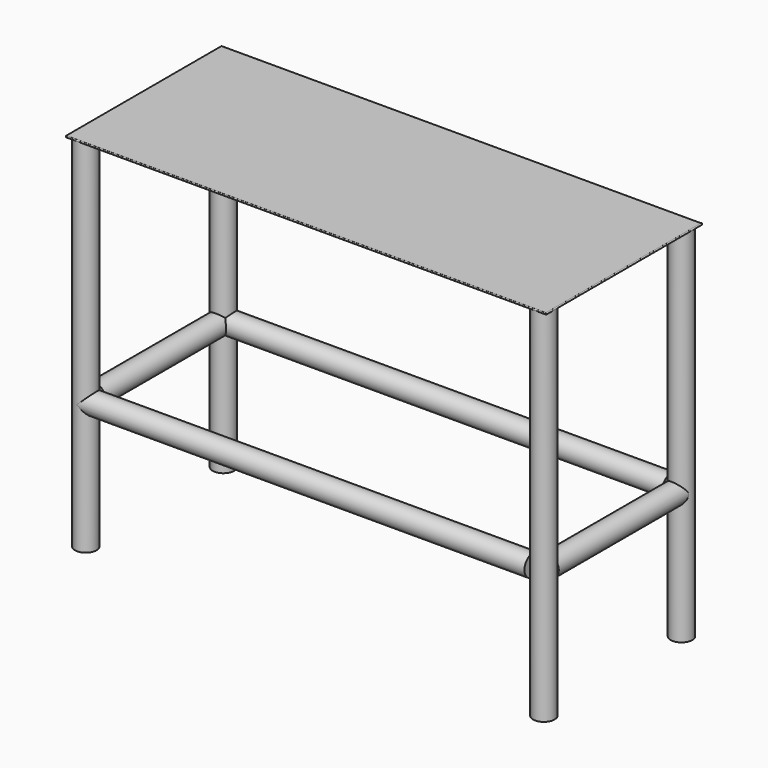
from build123d import *

# Parameters (mm, degrees)
F0_R          = 25
F1_DEPTH      = 840
F2_W          = 1115
F2_H          = 450
F3_DEPTH      = 3
F6_DEPTH      = 1115
F7_DEPTH      = 451.6069847541
F7_DEPTH_BACK = 1.6166657209
F9_R          = 25
F10_DEPTH     = 1039.876
F12_R         = 25
F13_DEPTH     = 1039.876
F15_R         = 25
F16_DEPTH     = 386.08
F18_R         = 25
F19_DEPTH     = 374.904


with BuildPart() as f1:
    # F0 (on Top) → F1 (new body)
    with BuildSketch(Plane.XY):
        with Locations((-532.5, 200)):
            Circle(F0_R)
    extrude(amount=F1_DEPTH)

    # F2 (on face) → F3 (join)
    with BuildSketch(Plane.XY.offset(840)):
        Rectangle(F2_W, F2_H)
    extrude(amount=F3_DEPTH)

    # F4 (on face) → F6 (join, through all)
    with BuildSketch(Plane(origin=(-557.5, 0, 0), x_dir=(0, -1, 0), z_dir=(-1, 0, 0))):
        with BuildLine():
            Line((-225, 840), (-225, 843))
            ThreePointArc((-225, 843), (-226.7016462617, 841.9811065332), (-226.6069847541, 840))
            Line((-226.6069847541, 840), (-225, 840))
        make_face()
        with BuildLine():
            Line((225, 840), (226.6166657209, 840))
            ThreePointArc((226.6166657209, 840), (226.7039372093, 841.9826309501), (225, 843))
            Line((225, 843), (225, 840))
        make_face()
    extrude(amount=-F6_DEPTH)

    # F5 (on face) → F7 (join, two sides)
    with BuildSketch(Plane.XZ.offset(225)) as f7_sk:
        with BuildLine():
            Line((557.5, 840), (559.1069847541, 840))
            ThreePointArc((559.1069847541, 840), (559.2016462617, 841.9811065332), (557.5, 843))
            Line((557.5, 843), (557.5, 840))
        make_face()
    extrude(amount=-F7_DEPTH)
    extrude(f7_sk.sketch, amount=F7_DEPTH_BACK)

    # F12 (on face) → F13 (join)
    with BuildSketch(Plane.YZ.offset(-532.5)):
        with Locations((200.4963755608, 300)):
            Circle(F12_R)
    extrude(amount=F13_DEPTH)

    # F18 (on face) → F19 (join)
    with BuildSketch(Plane(origin=(0, 200, 0), x_dir=(-1, 0, 0), z_dir=(0, 1, 0))):
        with Locations((532.0531129837, 300)):
            Circle(F18_R)
    extrude(amount=-F19_DEPTH)


with BuildPart() as f1b:
    # F0 (on Top) → F1, piece 2 (new body)
    with BuildSketch(Plane.XY):
        with Locations((-532.5, -200)):
            Circle(F0_R)
    extrude(amount=F1_DEPTH)

    # F9 (on face) → F10 (join)
    with BuildSketch(Plane.YZ.offset(-532.5)):
        with Locations((-200.0687867403, 300)):
            Circle(F9_R)
    extrude(amount=F10_DEPTH)


with BuildPart() as f1c:
    # F0 (on Top) → F1, piece 3 (new body)
    with BuildSketch(Plane.XY):
        with Locations((532.5, 200)):
            Circle(F0_R)
    extrude(amount=F1_DEPTH)

    # F15 (on face) → F16 (join)
    with BuildSketch(Plane(origin=(0, 200, 0), x_dir=(-1, 0, 0), z_dir=(0, 1, 0))):
        with Locations((-531.0813188553, 300)):
            Circle(F15_R)
    extrude(amount=-F16_DEPTH)


with BuildPart() as f1d:
    # F0 (on Top) → F1, piece 4 (new body)
    with BuildSketch(Plane.XY):
        with Locations((532.5, -200)):
            Circle(F0_R)
    extrude(amount=F1_DEPTH)


solid = Compound([f1.part, f1b.part, f1c.part, f1d.part])
